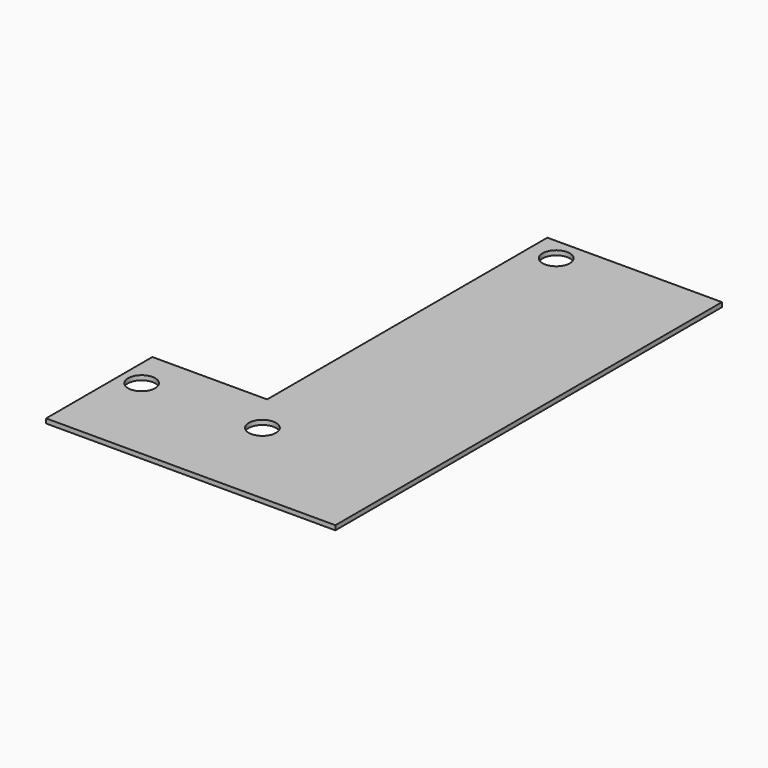
from build123d import *

# Parameters (mm, degrees)
F0_R     = 14.2875
F0_W     = 82.55
F0_H     = 368.3
F1_DEPTH = 4.7625


# Not quite as in the source:
# - a feature names something its author has since deleted; it is built from what else it names


with BuildPart() as f1:
    # F0 (on Top) → F1 (new body)
    with BuildSketch(Plane.XY):
        Polygon((19.05, -114.3), (-101.6, -114.3), (-101.6, -254), (101.6, -254), (101.6, -114.3), align=None)
        with Locations((-79.375, -156.21)):
            Circle(F0_R, mode=Mode.SUBTRACT)
        with Locations((47.625, -156.21)):
            Circle(F0_R, mode=Mode.SUBTRACT)
        Polygon((202.565, 254), (101.6, 254), (101.6, -114.3), (101.6, -254), (202.565, -254), align=None)
        with Locations((60.325, 69.85)):
            Rectangle(F0_W, F0_H)
        with Locations((47.625, 229.87)):
            Circle(F0_R, mode=Mode.SUBTRACT)
    extrude(amount=F1_DEPTH)


solid = f1.part
